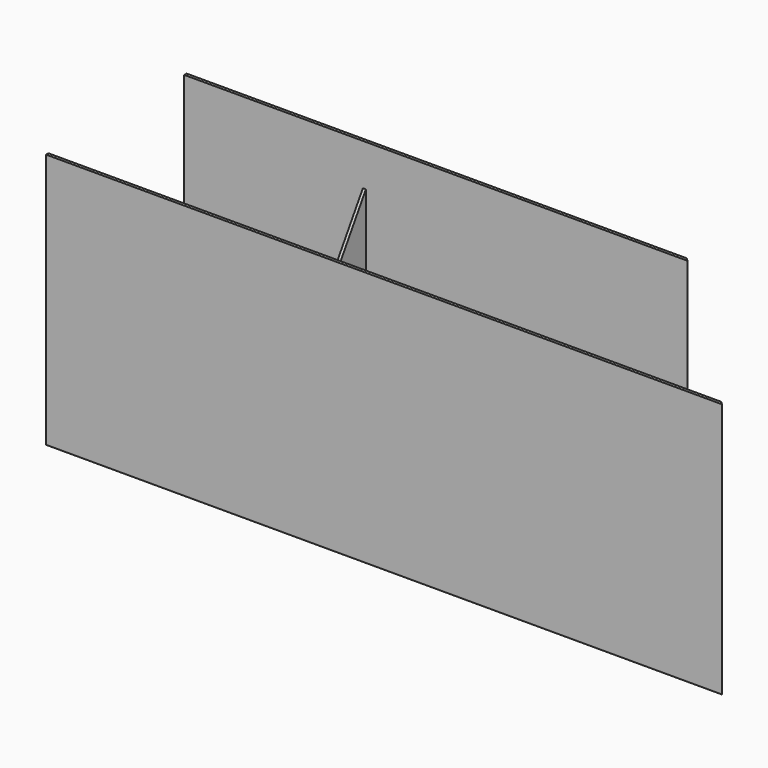
from build123d import *

# Parameters (mm, degrees)
F1_DEPTH = 1200
F4_DEPTH = 5
F5_W     = 1200
F5_H     = 230
F6_DEPTH = 4
F7_R     = 2
F9_DEPTH = 430.001


# Not quite as in the source:
# - a feature names something its author has since deleted; it is built from what else it names


with BuildPart() as f1:
    # F0 (on Right) → F1 (new body)
    with BuildSketch(Plane.YZ):
        Polygon((-295, 0), (0, 0), (0, 430), (-5, 430), (-5, 5), (-290, 5), (-290, 430), (-295, 430), align=None)
    extrude(amount=F1_DEPTH)



with BuildPart() as f4:
    # F3 (on offset) → F4 (new body)
    with BuildSketch(Plane.YZ.offset(300)):
        Polygon((-230, 0), (-5, 0), (-5, 360), align=None)
    extrude(amount=F4_DEPTH)


with BuildPart() as f1_1:
    add(f1.part)

    add(f4.part)  # F6 merges F4
    # F5 (on Top) → F6 (join)
    with BuildSketch(Plane.XY):
        with Locations((600, -115)):
            Rectangle(F5_W, F5_H)
    extrude(amount=F6_DEPTH)

    # F7
    f7_edges = [f1_1.edges().sort_by_distance(p)[0] for p in [
        (600, 0, 0),
        (600, -295, 0),
    ]]
    fillet(f7_edges, radius=F7_R)

    # F8 (on face) → F9 (cut, through all)
    with BuildSketch(Plane.XY.offset(430)):
        Polygon((840, 0), (1135, -295), (1200, -295), (1200, 0), align=None)
    extrude(amount=-F9_DEPTH, mode=Mode.SUBTRACT)


solid = f1_1.part
